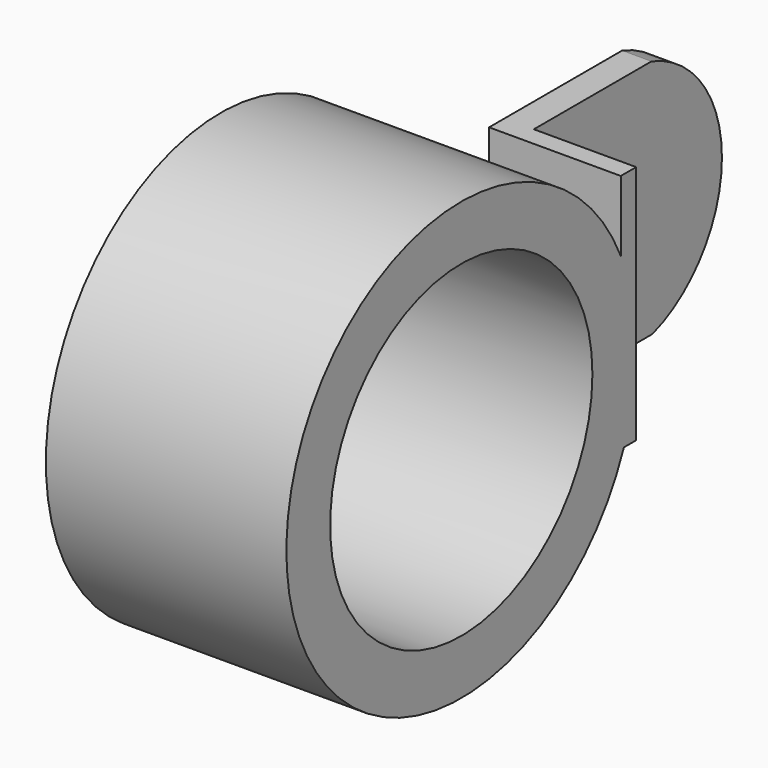
from build123d import *

# Parameters (mm, degrees)
F1_DEPTH = 25
F3_DEPTH = 25
F4_R     = 22.7224143994
F4_R_2   = 17.0375954798
F5_DEPTH = 25


# Not quite as in the source:
# - ends of sketch curves that miss each other by under 0.0002 mm in the source are joined


with BuildPart() as f1:
    # F0 (on Top) → F1 (new body)
    with BuildSketch(Plane.XY):
        Polygon((0, 0), (-10.6365969405, 0), (-10.6365969405, 24.4365315884), (-13.6861931533, 24.4365315884), (-13.6861931533, 0), (-13.6861931533, -2), (0, -2), align=None)
    extrude(amount=F1_DEPTH)

    # F2 (on face) → F3 (cut)
    with BuildSketch(Plane.YZ.offset(-10.6365969405)):
        with BuildLine():
            ThreePointArc((24.4365498995, 12.4780622919), (21.9456846424, 4.7798806359), (15.4173501195, 0))
            Line((15.4173501195, 0), (24.4365315884, 0))
            Line((24.4365315884, 0), (24.4365498995, 12.4780622919))
        make_face()
        with BuildLine():
            ThreePointArc((15.2820812933, 25), (21.9038763933, 20.233757287), (24.4365498995, 12.4780622919))
            Line((24.4365498995, 12.4780622919), (24.4365315884, 25))
            Line((24.4365315884, 25), (15.2820812933, 25))
        make_face()
    extrude(amount=-F3_DEPTH, mode=Mode.SUBTRACT)

    # F4 (on Right) → F5 (join)
    with BuildSketch(Plane.YZ):
        with Locations((-22.7224143994, 8.3613144234)):
            Circle(F4_R)
        with Locations((-22.7224143994, 8.3613144234)):
            Circle(F4_R_2, mode=Mode.SUBTRACT)
    extrude(amount=-F5_DEPTH)


solid = f1.part
